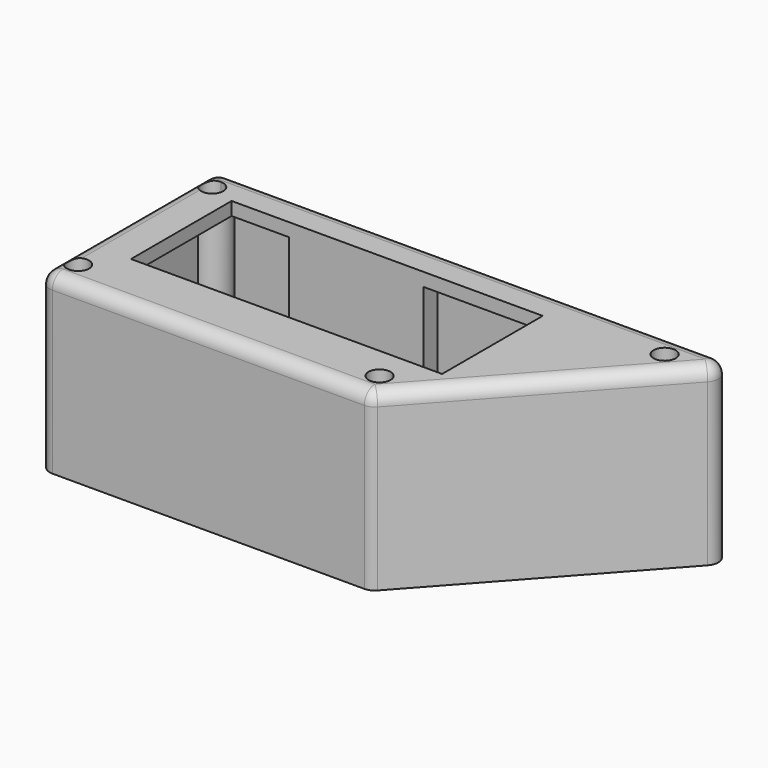
from build123d import *

# Parameters (mm, degrees)
F1_DEPTH     = 3
F0_R         = 2.5
F0_W         = 30.5
F0_H         = 9.5
F0_H_2       = 4
F2_DEPTH     = 39.6
F3_T1_DEPTH  = 70.6639127859
F3_T3_DEPTH  = 44.1
F3_T5_DEPTH  = 39.9402180353
F3_T7_DEPTH  = 59.1959458071
F3_T9_DEPTH  = 53.4402180353
F3_T11_DEPTH = 110.2639127859
F3_T13_DEPTH = 44
F3_S17_W     = 3
F3_S17_H     = 3
F3_T18_DEPTH = 3
F3_T24_DEPTH = 3
F3_T30_DEPTH = 3
F3_S35_W     = 3
F3_S35_H     = 3
F3_T36_DEPTH = 3


# Not quite as in the source:
# - a fillet or chamfer that OpenCascade refuses, or shapes differently, is made with other operations: its cross-section is extruded or revolved along the edge and cut away or added


with BuildPart() as f1:
    # F0 (on Top) → F1 (new body)
    with BuildSketch(Plane.XY):
        with BuildLine():
            Line((10, -36.5), (10, -8))
            Line((10, -8), (23, -8))
            Line((23, -8), (23, -4))
            Line((23, -4), (7.4641016151, -4))
            ThreePointArc((7.4641016151, -4), (7.4641016151, -8), (4, -10))
            Line((4, -10), (4, -40))
            ThreePointArc((4, -40), (7.4641016151, -42), (7.4641016151, -46))
            Line((7.4641016151, -46), (23, -46))
            Line((23, -46), (23, -36.5))
            Line((23, -36.5), (10, -36.5))
        make_face()
    extrude(amount=-F1_DEPTH)



with BuildPart() as f1b:
    # F0 (on Top) → F1, piece 2 (new body)
    with BuildSketch(Plane.XY):
        with BuildLine():
            Line((53.5, -4), (53.5, -8))
            Line((53.5, -8), (80.5, -8))
            Line((80.5, -8), (80.5, -36.5))
            Line((80.5, -36.5), (53.5, -36.5))
            Line((53.5, -36.5), (53.5, -46))
            Line((53.5, -46), (68.8637239566, -46))
            ThreePointArc((68.8637239566, -46), (70.700471232, -40.3459997464), (76.1317756715, -42.7630830107))
            Line((76.1317756715, -42.7630830107), (105.697052057, -9.9127759158))
            ThreePointArc((105.697052057, -9.9127759158), (102.8738253182, -7.6273543397), (103.0637239566, -4))
            Line((103.0637239566, -4), (53.5, -4))
        make_face()
    extrude(amount=-F1_DEPTH)


with BuildPart() as f1_1:
    add(f1.part)

    add(f1b.part)  # F2 merges F1b
    # F0 (on Top) → F2 (join)
    with BuildSketch(Plane.XY):
        Polygon((120, 0), (0, 0), (0, -50), (75, -50), align=None)
        with BuildLine():
            ThreePointArc((4, -46.5), (2.232233047, -42.232233047), (6.5, -44))
            ThreePointArc((6.5, -44), (5.767766953, -45.767766953), (4, -46.5))
        make_face(mode=Mode.SUBTRACT)
        with BuildLine():
            Line((7.4641016151, -4), (23, -4))
            Line((23, -4), (53.5, -4))
            Line((53.5, -4), (103.0637239566, -4))
            ThreePointArc((103.0637239566, -4), (102.8738253182, -7.6273543397), (105.697052057, -9.9127759158))
            Line((105.697052057, -9.9127759158), (76.1317756715, -42.7630830107))
            ThreePointArc((76.1317756715, -42.7630830107), (70.700471232, -40.3459997464), (68.8637239566, -46))
            Line((68.8637239566, -46), (53.5, -46))
            Line((53.5, -46), (23, -46))
            Line((23, -46), (7.4641016151, -46))
            ThreePointArc((7.4641016151, -46), (7.4641016151, -42), (4, -40))
            Line((4, -40), (4, -10))
            ThreePointArc((4, -10), (7.4641016151, -8), (7.4641016151, -4))
        make_face(mode=Mode.SUBTRACT)
        with Locations((72.3278255718, -44)):
            Circle(F0_R, mode=Mode.SUBTRACT)
        with BuildLine():
            ThreePointArc((4, -3.5), (5.767766953, -4.232233047), (6.5, -6))
            ThreePointArc((6.5, -6), (2.232233047, -7.767766953), (4, -3.5))
        make_face(mode=Mode.SUBTRACT)
        with Locations((106.5278255718, -6)):
            Circle(F0_R, mode=Mode.SUBTRACT)
        with Locations((38.25, -41.25)):
            Rectangle(F0_W, F0_H)
        with Locations((38.25, -6)):
            Rectangle(F0_W, F0_H_2)
    extrude(amount=-F2_DEPTH)

    # F3: fillet of radius 3 on 8 edges, made by hand

    # F3_s2 → F3_t1 (cut)
    with BuildSketch(Plane.YZ.offset(3)):
        with BuildLine():
            ThreePointArc((-50, -3), (-49.1213203436, -0.8786796564), (-47, 0))
            Line((-47, 0), (-50, 0))
            Line((-50, 0), (-50, -3))
        make_face()
    extrude(amount=F3_T1_DEPTH, mode=Mode.SUBTRACT)

    # F3_s4 → F3_t3 (cut)
    with BuildSketch(Plane.XY.offset(-47.1)):
        with BuildLine():
            ThreePointArc((3, -50), (0.8786796564, -49.1213203436), (0, -47))
            Line((0, -47), (0, -50))
            Line((0, -50), (3, -50))
        make_face()
        with BuildLine():
            ThreePointArc((0, -3), (0.8786796564, -0.8786796564), (3, 0))
            Line((3, 0), (0, 0))
            Line((0, 0), (0, -3))
        make_face()
    extrude(amount=F3_T3_DEPTH, mode=Mode.SUBTRACT)

    # F3_s6 → F3_t5 (cut)
    with BuildSketch(Plane.XY.offset(-42.9402180353)):
        with BuildLine():
            ThreePointArc((75.8937952246, -49.0068941949), (74.8844285407, -49.7405001902), (73.6639127859, -50))
            Line((73.6639127859, -50), (75, -50))
            Line((75, -50), (75.8937952246, -49.0068941949))
        make_face()
    extrude(amount=F3_T5_DEPTH, mode=Mode.SUBTRACT)

    # F3_s8 → F3_t7 (cut)
    with BuildSketch(Plane(origin=(9.5954526832, 10.6616140924, 0), x_dir=(0, 0, 1), z_dir=(0.6689647316, 0.7432941462, 0))):
        with BuildLine():
            ThreePointArc((-3, 89.1952975497), (-0.8786796564, 88.3166178932), (0, 86.1952975497))
            Line((0, 86.1952975497), (0, 89.1952975497))
            Line((0, 89.1952975497), (-3, 89.1952975497))
        make_face()
    extrude(amount=F3_T7_DEPTH, mode=Mode.SUBTRACT)

    # F3_s10 → F3_t9 (cut)
    with BuildSketch(Plane.XY.offset(-56.4402180353)):
        with BuildLine():
            ThreePointArc((115.4937952246, -5.0068941949), (116.004412976, -1.7794842452), (113.2639127859, 0))
            Line((113.2639127859, 0), (120, 0))
            Line((120, 0), (115.4937952246, -5.0068941949))
        make_face()
    extrude(amount=F3_T9_DEPTH, mode=Mode.SUBTRACT)

    # F3_s12 → F3_t11 (cut)
    with BuildSketch(Plane.YZ.offset(3)):
        with BuildLine():
            ThreePointArc((0, -3), (-0.8786796564, -0.8786796564), (-3, 0))
            Line((-3, 0), (0, 0))
            Line((0, 0), (0, -3))
        make_face()
    extrude(amount=F3_T11_DEPTH, mode=Mode.SUBTRACT)

    # F3_s14 → F3_t13 (cut)
    with BuildSketch(Plane.XZ.offset(3)):
        with BuildLine():
            ThreePointArc((0, -3), (0.8786796564, -0.8786796564), (3, 0))
            Line((3, 0), (0, 0))
            Line((0, 0), (0, -3))
        make_face()
    extrude(amount=F3_T13_DEPTH, mode=Mode.SUBTRACT)


with BuildPart() as f3_tool16:
    # F3_s17 → F3_t18 (new body)
    with BuildSketch(Plane.XY.offset(-3)):
        with Locations((1.5, -48.5)):
            Rectangle(F3_S17_W, F3_S17_H)
    extrude(amount=F3_T18_DEPTH)

    # F3_s19 → F3_t20 (revolve, cut)
    with BuildSketch(Plane(origin=(3, -47, -3), x_dir=(0.7071067812, 0.7071067812, 0), z_dir=(0.7071067812, -0.7071067812, 0))):
        with BuildLine():
            ThreePointArc((0, -3), (3, 0), (0, 3))
            Line((0, 3), (0, -3))
        make_face()
    revolve(axis=Axis((3, -47, -3), (0, 0, 1)), mode=Mode.SUBTRACT)


with BuildPart() as f1_2:
    add(f1_1.part)

    # F3_t15: cut F3_tool16
    add(f3_tool16.part, mode=Mode.SUBTRACT)


with BuildPart() as f3_tool22:
    # F3_s23 → F3_t24 (new body)
    with BuildSketch(Plane.XY.offset(-3)):
        Polygon((73.6639127859, -47), (75.8937952246, -49.0068941949), (75, -50), (73.6639127859, -50), align=None)
    extrude(amount=F3_T24_DEPTH)

    # F3_s25 → F3_t26 (revolve, cut)
    with BuildSketch(Plane(origin=(73.6639127859, -47, -3), x_dir=(-0.4068385849, 0.9135000634, 0), z_dir=(0.9135000634, 0.4068385849, 0))):
        with BuildLine():
            ThreePointArc((0, -3), (3, 0), (0, 3))
            Line((0, 3), (0, -3))
        make_face()
    revolve(axis=Axis((73.6639127859, -47, -3), (0, 0, 1)), mode=Mode.SUBTRACT)


with BuildPart() as f1_3:
    add(f1_2.part)

    # F3_t21: cut F3_tool22
    add(f3_tool22.part, mode=Mode.SUBTRACT)


with BuildPart() as f3_tool28:
    # F3_s29 → F3_t30 (new body)
    with BuildSketch(Plane.XY.offset(-3)):
        Polygon((113.2639127859, -3), (115.4937952246, -5.0068941949), (120, 0), (113.2639127859, 0), align=None)
    extrude(amount=F3_T30_DEPTH)

    # F3_s31 → F3_t32 (revolve, cut)
    with BuildSketch(Plane(origin=(113.2639127859, -3, -3), x_dir=(-0.9135000634, -0.4068385849, 0), z_dir=(-0.4068385849, 0.9135000634, 0))):
        with BuildLine():
            ThreePointArc((0, -3), (3, 0), (0, 3))
            Line((0, 3), (0, -3))
        make_face()
    revolve(axis=Axis((113.2639127859, -3, -3), (0, 0, 1)), mode=Mode.SUBTRACT)


with BuildPart() as f1_4:
    add(f1_3.part)

    # F3_t27: cut F3_tool28
    add(f3_tool28.part, mode=Mode.SUBTRACT)


with BuildPart() as f3_tool34:
    # F3_s35 → F3_t36 (new body)
    with BuildSketch(Plane.XZ.offset(3)):
        with Locations((1.5, -1.5)):
            Rectangle(F3_S35_W, F3_S35_H)
    extrude(amount=-F3_T36_DEPTH)

    # F3_s37 → F3_t38 (revolve, cut)
    with BuildSketch(Plane(origin=(3, -3, -3), x_dir=(0.7071067812, 0, -0.7071067812), z_dir=(0.7071067812, 0, 0.7071067812))):
        with BuildLine():
            ThreePointArc((0, -3), (3, 0), (0, 3))
            Line((0, 3), (0, -3))
        make_face()
    revolve(axis=Axis((3, -3, -3), (0, 1, 0)), mode=Mode.SUBTRACT)


with BuildPart() as f1_5:
    add(f1_4.part)

    # F3_t33: cut F3_tool34
    add(f3_tool34.part, mode=Mode.SUBTRACT)


solid = f1_5.part
